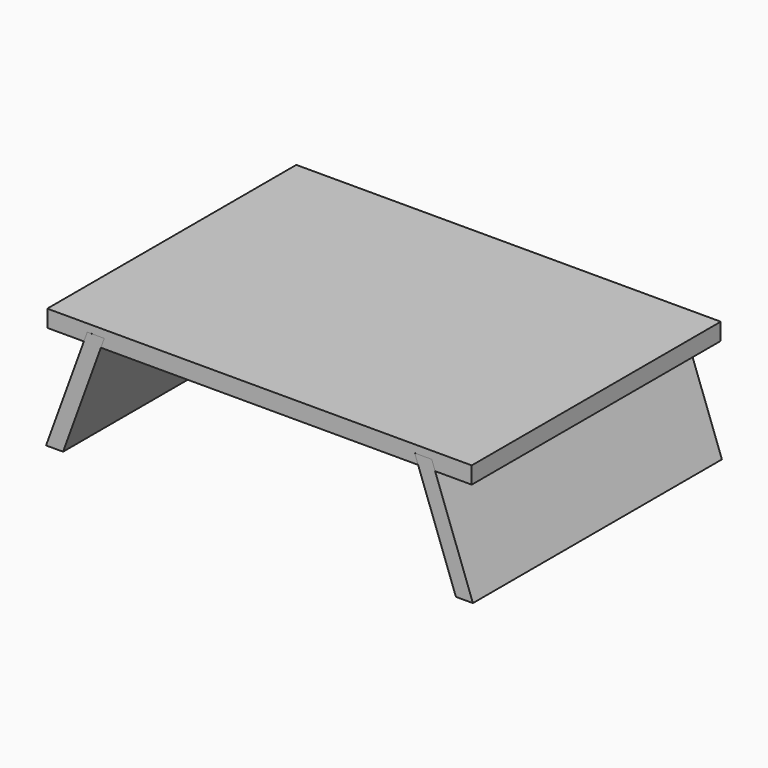
from build123d import *

# Parameters (mm, degrees)
F0_W     = 300
F0_H     = 220
F1_DEPTH = 12
F3_DEPTH = 220
F4_ANGLE = -20


# Not quite as in the source:
# - a feature names something its author has since deleted; it is built from what else it names


with BuildPart() as f1:
    # F0 (on Top) → F1 (new body)
    with BuildSketch(Plane.XY):
        Rectangle(F0_W, F0_H)
    extrude(amount=F1_DEPTH)



with BuildPart() as f3:
    # F2 (on Front) → F3 (new body)
    with BuildSketch(Plane.XZ):
        Polygon((90.735743386, -85.723820842), (102.0120548354, -89.8280625619), (102.0120548354, -4.6938407638), (90.735743386, -0.5895990439), align=None)
    extrude(amount=F3_DEPTH)


with BuildPart() as f3_1:
    # F4: moved
    add(f3.part.rotate(Axis((90.735743386, -110, -85.723820842), (0, 1, 0)), F4_ANGLE))


with BuildPart() as f3_2:
    # F5: moved
    add(f3_1.part.moved(Location((48.1, 109.99, 12.3))))


with BuildPart() as f1_1:
    add(f1.part)

    add(f3_2.part)  # F6 merges F3
    # F6: F3 across plane
    add(f3_2.part.mirror(Plane.YZ))


solid = f1_1.part
